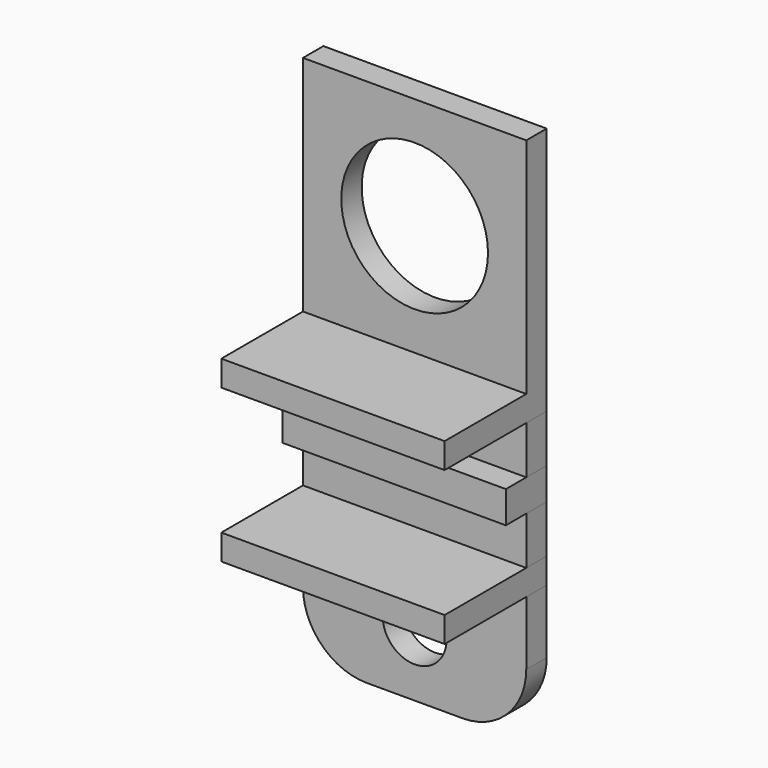
from build123d import *

# Parameters (mm, degrees)
F0_W     = 35
F0_H     = 35
F0_R     = 11.5
F1_DEPTH = 4
F0_H_2   = 7.5
F0_R_2   = 5
F0_H_3   = 4
F2_DEPTH = 20
F0_H_4   = 5
F3_DEPTH = 8


with BuildPart() as f1:
    # F0 (on Front) → F1 (new body)
    with BuildSketch(Plane.XZ):
        with Locations((105, 17.5)):
            Rectangle(F0_W, F0_H)
        with Locations((105, 17.5)):
            Circle(F0_R, mode=Mode.SUBTRACT)
    extrude(amount=F1_DEPTH)

    # F0 (on Front) → F2 (join)
    with BuildSketch(Plane.XZ):
        with Locations((105, -2)):
            Rectangle(F0_W, F0_H_3)
    extrude(amount=F2_DEPTH)


with BuildPart() as f1b:
    # F0 (on Front) → F1, piece 2 (new body)
    with BuildSketch(Plane.XZ):
        with Locations((105, -7.75)):
            Rectangle(F0_W, F0_H_2)
    extrude(amount=F1_DEPTH)


with BuildPart() as f1c:
    # F0 (on Front) → F1, piece 3 (new body)
    with BuildSketch(Plane.XZ):
        with Locations((105, -20.25)):
            Rectangle(F0_W, F0_H_2)
    extrude(amount=F1_DEPTH)


with BuildPart() as f1d:
    # F0 (on Front) → F1, piece 4 (new body)
    with BuildSketch(Plane.XZ):
        with BuildLine():
            Line((122.5, -28), (87.5, -28))
            Line((87.5, -28), (87.5, -38))
            ThreePointArc((87.5, -38), (90.4289321881, -45.0710678119), (97.5, -48))
            Line((97.5, -48), (112.5, -48))
            ThreePointArc((112.5, -48), (119.5710678119, -45.0710678119), (122.5, -38))
            Line((122.5, -38), (122.5, -28))
        make_face()
        with Locations((105, -38)):
            Circle(F0_R_2, mode=Mode.SUBTRACT)
    extrude(amount=F1_DEPTH)


with BuildPart() as f2:
    # F0 (on Front) → F2, piece 2 (new body)
    with BuildSketch(Plane.XZ):
        with Locations((105, -26)):
            Rectangle(F0_W, F0_H_3)
    extrude(amount=F2_DEPTH)


with BuildPart() as f3:
    # F0 (on Front) → F3 (new body)
    with BuildSketch(Plane.XZ):
        with Locations((105, -14)):
            Rectangle(F0_W, F0_H_4)
    extrude(amount=F3_DEPTH)


solid = Compound([f1.part, f1b.part, f1c.part, f1d.part, f2.part, f3.part])
